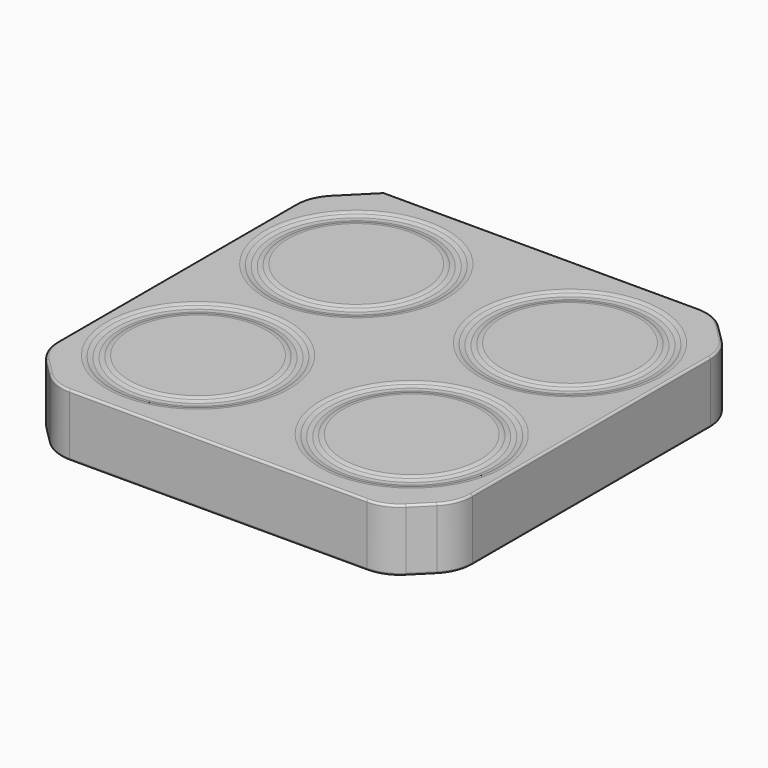
from build123d import *

# Parameters (mm, degrees)
F0_W     = 50.8
F0_H     = 50.8
F1_DEPTH = 7.62
F2_R     = 10.4028290025
F2_R_2   = 9.1328290025
F3_DEPTH = 0.254
F4_SIZE  = 5.08
F6_R     = 1.27
F7_R     = 5.08
F8_R     = 5.08
F9_R     = 0.254


# Not quite as in the source:
# - a fillet or chamfer that OpenCascade refuses, or shapes differently, is made with other operations: its cross-section is extruded or revolved along the edge and cut away or added


with BuildPart() as f1:
    # F0 (on Top) → F1 (new body)
    with BuildSketch(Plane.XY):
        Rectangle(F0_W, F0_H)
    extrude(amount=F1_DEPTH)

    # F2 (on face) → F3 (cut)
    with BuildSketch(Plane.XY.offset(7.62)):
        with Locations((-13.0905816332, 12.1185639873)):
            Circle(F2_R)
        with Locations((-13.0905816332, 12.1185639873)):
            Circle(F2_R_2, mode=Mode.SUBTRACT)
        with Locations((13.0905816332, 12.1185639873)):
            Circle(F2_R)
        with Locations((13.0905816332, 12.1185639873)):
            Circle(F2_R_2, mode=Mode.SUBTRACT)
        with Locations((-13.0905816332, -12.1185639873)):
            Circle(F2_R)
        with Locations((-13.0905816332, -12.1185639873)):
            Circle(F2_R_2, mode=Mode.SUBTRACT)
        with Locations((13.0905816332, -12.1185639873)):
            Circle(F2_R)
        with Locations((13.0905816332, -12.1185639873)):
            Circle(F2_R_2, mode=Mode.SUBTRACT)
    extrude(amount=-F3_DEPTH, mode=Mode.SUBTRACT)

    # F4
    f4_edges = [f1.edges().sort_by_distance(p)[0] for p in [
        (-25.4, -25.4, 3.81),
        (25.4, -25.4, 3.81),
        (-25.4, 25.4, 3.81),
        (25.4, 25.4, 3.81),
    ]]
    chamfer(f4_edges, length=F4_SIZE)

    # F5: fillet of radius 1.27 on 8 edges, made by hand

    # F5_s1 → F5_t2 (revolve, cut)
    with BuildSketch(Plane.XZ.offset(-12.1185639873)):
        with BuildLine():
            ThreePointArc((-3.9577526306, 7.366), (-4.3181433678, 7.5548277885), (-4.7197526306, 7.62))
            Line((-4.7197526306, 7.62), (-3.9577526306, 7.62))
            Line((-3.9577526306, 7.62), (-3.9577526306, 7.366))
        make_face()
    revolve(axis=Axis((-13.0905816332, 12.1185639873, 7.62), (0, 0, 1)), mode=Mode.SUBTRACT)

    # F5_s3 → F5_t4 (revolve, cut)
    with BuildSketch(Plane.XZ.offset(-12.1185639873)):
        with BuildLine():
            ThreePointArc((-1.9257526306, 7.62), (-2.3273618935, 7.5548277885), (-2.6877526306, 7.366))
            Line((-2.6877526306, 7.366), (-2.6877526306, 7.62))
            Line((-2.6877526306, 7.62), (-1.9257526306, 7.62))
        make_face()
    revolve(axis=Axis((-13.0905816332, 12.1185639873, 7.62), (0, 0, 1)), mode=Mode.SUBTRACT)

    # F5_s5 → F5_t6 (revolve, cut)
    with BuildSketch(Plane.XZ.offset(-12.1185639873)):
        with BuildLine():
            ThreePointArc((24.2554106357, 7.62), (23.8538013728, 7.5548277885), (23.4934106357, 7.366))
            Line((23.4934106357, 7.366), (23.4934106357, 7.62))
            Line((23.4934106357, 7.62), (24.2554106357, 7.62))
        make_face()
    revolve(axis=Axis((13.0905816332, 12.1185639873, 7.62), (0, 0, 1)), mode=Mode.SUBTRACT)

    # F5_s7 → F5_t8 (revolve, cut)
    with BuildSketch(Plane.XZ.offset(-12.1185639873)):
        with BuildLine():
            ThreePointArc((22.2234106357, 7.366), (21.8630198985, 7.5548277885), (21.4614106357, 7.62))
            Line((21.4614106357, 7.62), (22.2234106357, 7.62))
            Line((22.2234106357, 7.62), (22.2234106357, 7.366))
        make_face()
    revolve(axis=Axis((13.0905816332, 12.1185639873, 7.62), (0, 0, 1)), mode=Mode.SUBTRACT)

    # F5_s9 → F5_t10 (revolve, cut)
    with BuildSketch(Plane.XZ.offset(12.1185639873)):
        with BuildLine():
            ThreePointArc((24.2554106357, 7.62), (23.8538013728, 7.5548277885), (23.4934106357, 7.366))
            Line((23.4934106357, 7.366), (23.4934106357, 7.62))
            Line((23.4934106357, 7.62), (24.2554106357, 7.62))
        make_face()
    revolve(axis=Axis((13.0905816332, -12.1185639873, 7.62), (0, 0, 1)), mode=Mode.SUBTRACT)

    # F5_s11 → F5_t12 (revolve, cut)
    with BuildSketch(Plane.XZ.offset(12.1185639873)):
        with BuildLine():
            ThreePointArc((22.2234106357, 7.366), (21.8630198985, 7.5548277885), (21.4614106357, 7.62))
            Line((21.4614106357, 7.62), (22.2234106357, 7.62))
            Line((22.2234106357, 7.62), (22.2234106357, 7.366))
        make_face()
    revolve(axis=Axis((13.0905816332, -12.1185639873, 7.62), (0, 0, 1)), mode=Mode.SUBTRACT)

    # F5_s13 → F5_t14 (revolve, cut)
    with BuildSketch(Plane.XZ.offset(12.1185639873)):
        with BuildLine():
            ThreePointArc((-3.9577526306, 7.366), (-4.3181433678, 7.5548277885), (-4.7197526306, 7.62))
            Line((-4.7197526306, 7.62), (-3.9577526306, 7.62))
            Line((-3.9577526306, 7.62), (-3.9577526306, 7.366))
        make_face()
    revolve(axis=Axis((-13.0905816332, -12.1185639873, 7.62), (0, 0, 1)), mode=Mode.SUBTRACT)

    # F5_s15 → F5_t16 (revolve, cut)
    with BuildSketch(Plane.XZ.offset(12.1185639873)):
        with BuildLine():
            ThreePointArc((-1.9257526306, 7.62), (-2.3273618935, 7.5548277885), (-2.6877526306, 7.366))
            Line((-2.6877526306, 7.366), (-2.6877526306, 7.62))
            Line((-2.6877526306, 7.62), (-1.9257526306, 7.62))
        make_face()
    revolve(axis=Axis((-13.0905816332, -12.1185639873, 7.62), (0, 0, 1)), mode=Mode.SUBTRACT)

    # F6
    f6_edges = [f1.edges().sort_by_distance(p)[0] for p in [
        (-23.493411, 12.118564, 7.366),
        (-22.223411, 12.118564, 7.366),
        (2.687753, 12.118564, 7.366),
        (3.957753, 12.118564, 7.366),
        (-22.223411, -12.118564, 7.366),
        (2.687753, -12.118564, 7.366),
        (3.957753, -12.118564, 7.366),
        (-23.493411, -12.118564, 7.366),
    ]]
    fillet(f6_edges, radius=F6_R)

    # F7
    f7_edges = [f1.edges().sort_by_distance(p)[0] for p in [
        (-25.4, -20.32, 3.81),
        (-20.32, -25.4, 3.81),
    ]]
    fillet(f7_edges, radius=F7_R)

    # F8
    f8_edges = [f1.edges().sort_by_distance(p)[0] for p in [
        (-25.4, 20.32, 3.81),
        (20.32, -25.4, 3.81),
        (25.4, -20.32, 3.81),
        (25.4, 20.32, 3.81),
        (20.32, 25.4, 3.81),
    ]]
    fillet(f8_edges, radius=F8_R)

    # F9
    f9_edges = [f1.edges().sort_by_distance(p)[0] for p in [
        (0, -25.4, 0),
        (-22.86, -22.86, 7.62),
        (-25.4, 0, 7.62),
        (-25.013308, 20.159827, 7.62),
        (-25.013308, -20.159827, 7.62),
        (-22.116051, 23.603949, 7.62),
        (-1.052102, 25.4, 7.62),
        (-20.159827, -25.013308, 7.62),
        (20.159827, 25.013308, 7.62),
        (0, -25.4, 7.62),
        (22.86, 22.86, 7.62),
        (20.159827, -25.013308, 7.62),
        (25.013308, 20.159827, 7.62),
        (22.86, -22.86, 7.62),
        (25.4, 0, 7.62),
        (25.013308, -20.159827, 7.62),
        (-25.4, 0, 0),
        (-25.013308, 20.159827, 0),
        (-25.013308, -20.159827, 0),
        (-22.116051, 23.603949, 0),
        (-22.86, -22.86, 0),
        (-1.052102, 25.4, 0),
        (-20.159827, -25.013308, 0),
        (20.159827, 25.013308, 0),
        (22.86, 22.86, 0),
        (20.159827, -25.013308, 0),
        (25.013308, 20.159827, 0),
        (22.86, -22.86, 0),
        (25.4, 0, 0),
        (25.013308, -20.159827, 0),
    ]]
    fillet(f9_edges, radius=F9_R)


solid = f1.part
